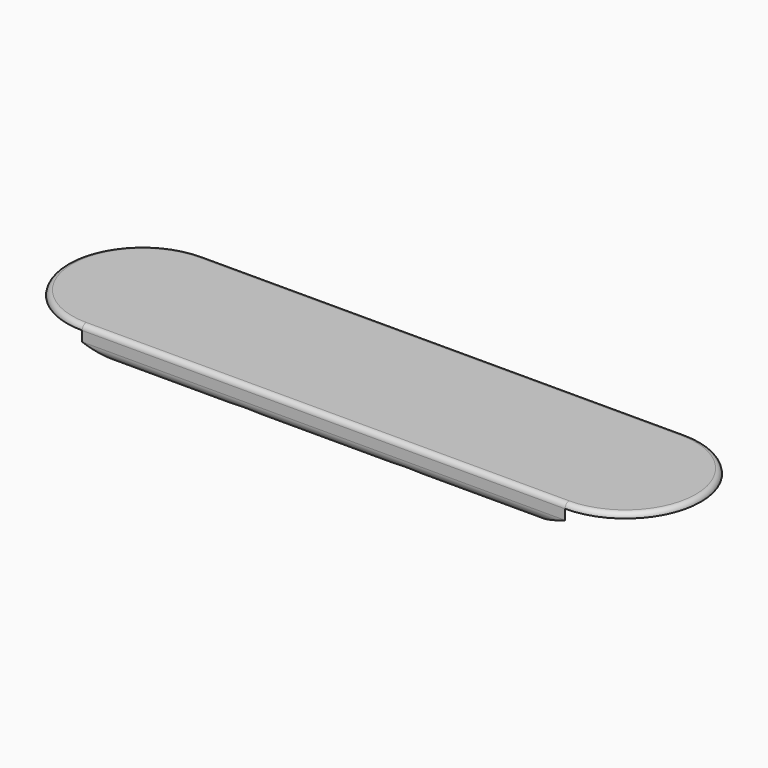
from build123d import *

# Parameters (mm, degrees)
F0_R        = 14.5
F1_DEPTH    = 5
F2_DEPTH    = 4
F3_T1_DEPTH = 113
F4_R        = 0.99999


# Not quite as in the source:
# - a fillet or chamfer that OpenCascade refuses, or shapes differently, is made with other operations: its cross-section is extruded or revolved along the edge and cut away or added
# - a fillet or chamfer is up to 0.001 mm smaller than in the source, because OpenCascade refuses the exact size


with BuildPart() as f1:
    # F0 (on Top) → F1 (new body)
    with BuildSketch(Plane.XY):
        with BuildLine():
            ThreePointArc((47, 0), (42.6066017178, 10.6066017178), (32, 15))
            ThreePointArc((32, 15), (17, 0), (32, -15))
            ThreePointArc((32, -15), (42.6066017178, -10.6066017178), (47, 0))
        make_face()
        with BuildLine():
            ThreePointArc((-64, 15), (-53.3933982822, 10.6066017178), (-49, 0))
            ThreePointArc((-49, 0), (-53.3933982822, -10.6066017178), (-64, -15))
            Line((-64, -15), (32, -15))
            ThreePointArc((32, -15), (17, 0), (32, 15))
            Line((32, 15), (-64, 15))
        make_face()
        with Locations((-32, 0)):
            Circle(F0_R, mode=Mode.SUBTRACT)
        Circle(F0_R, mode=Mode.SUBTRACT)
        Circle(F0_R)
        with Locations((-32, 0)):
            Circle(F0_R)
        with BuildLine():
            ThreePointArc((-64, -15), (-53.3933982822, -10.6066017178), (-49, 0))
            ThreePointArc((-49, 0), (-53.3933982822, 10.6066017178), (-64, 15))
            ThreePointArc((-64, 15), (-79, 0), (-64, -15))
        make_face()
    extrude(amount=F1_DEPTH)

    # F0 (on Top) → F2 (cut)
    with BuildSketch(Plane.XY):
        with BuildLine():
            ThreePointArc((47, 0), (42.6066017178, 10.6066017178), (32, 15))
            ThreePointArc((32, 15), (17, 0), (32, -15))
            ThreePointArc((32, -15), (42.6066017178, -10.6066017178), (47, 0))
        make_face()
        Circle(F0_R)
        with Locations((-32, 0)):
            Circle(F0_R)
        with BuildLine():
            ThreePointArc((-64, -15), (-53.3933982822, -10.6066017178), (-49, 0))
            ThreePointArc((-49, 0), (-53.3933982822, 10.6066017178), (-64, 15))
            ThreePointArc((-64, 15), (-79, 0), (-64, -15))
        make_face()
    extrude(amount=F2_DEPTH, mode=Mode.SUBTRACT)

    # F3: fillet of radius 2 on 2 edges, made by hand

    # F3_s2 → F3_t1 (cut)
    with BuildSketch(Plane.YZ.offset(-72.5)):
        with BuildLine():
            ThreePointArc((-13, 0), (-14.4142135624, 0.5857864376), (-15, 2))
            Line((-15, 2), (-15, 0))
            Line((-15, 0), (-13, 0))
        make_face()
        with BuildLine():
            ThreePointArc((15, 2), (14.4142135624, 0.5857864376), (13, 0))
            Line((13, 0), (15, 0))
            Line((15, 0), (15, 2))
        make_face()
    extrude(amount=F3_T1_DEPTH, mode=Mode.SUBTRACT)

    # F4 (radius 1 in the source; OpenCascade refuses exactly that, so slightly less here)
    f4_edges = [f1.edges().sort_by_distance(p)[0] for p in [
        (47, 0, 5),
        (-16, 15, 5),
        (-79, 0, 5),
        (-16, -15, 5),
    ]]
    fillet(f4_edges, radius=F4_R)


solid = f1.part
